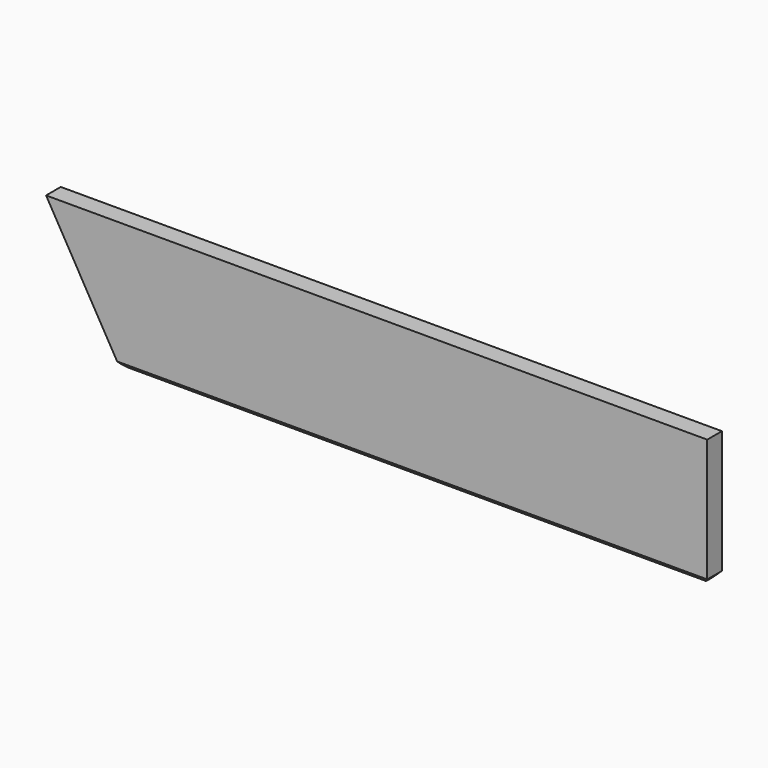
from build123d import *

# Parameters (mm, degrees)
F0_W        = 457.2
F0_H        = 88.9
F1_DEPTH    = 12.7
F3_DEPTH    = 12.701
F4_T1_DEPTH = 425.4697854373
F4_T3_DEPTH = 32.2962243683
F4_T5_DEPTH = 24.3646579033


# Not quite as in the source:
# - a fillet or chamfer that OpenCascade refuses, or shapes differently, is made with other operations: its cross-section is extruded or revolved along the edge and cut away or added
# - a feature names something its author has since deleted; it is built from what else it names


with BuildPart() as f1:
    # F0 (on Front) → F1 (new body)
    with BuildSketch(Plane.XZ):
        Rectangle(F0_W, F0_H)
    extrude(amount=F1_DEPTH)

    # F2 (on face) → F3 (cut, through all)
    with BuildSketch(Plane.XZ.offset(12.7)):
        Polygon((-177.273561069, -44.45), (-228.6, 44.45), (-228.6, -44.45), align=None)
    extrude(amount=-F3_DEPTH, mode=Mode.SUBTRACT)

    # F4: chamfer of 3.81 on 4 edges, made by hand

    # F4_s2 → F4_t1 (cut)
    with BuildSketch(Plane.YZ.offset(-187.0716732532)):
        Polygon((0, -40.64), (-3.81, -44.45), (0, -44.45), align=None)
        Polygon((-12.7, -40.64), (-8.89, -44.45), (-12.7, -44.45), align=None)
    extrude(amount=F4_T1_DEPTH, mode=Mode.SUBTRACT)

    # F4_s4 → F4_t3 (cut)
    with BuildSketch(Plane.XZ.offset(-9.7981121842)):
        Polygon((228.6, -40.64), (224.79, -44.45), (228.6, -44.45), align=None)
    extrude(amount=F4_T3_DEPTH, mode=Mode.SUBTRACT)

    # F4_s6 → F4_t5 (cut)
    with BuildSketch(Plane.XZ.offset(-5.8323289516)):
        Polygon((-178.3734133318, -42.545), (-175.0738565434, -44.45), (-177.273561069, -44.45), align=None)
    extrude(amount=F4_T5_DEPTH, mode=Mode.SUBTRACT)


solid = f1.part
